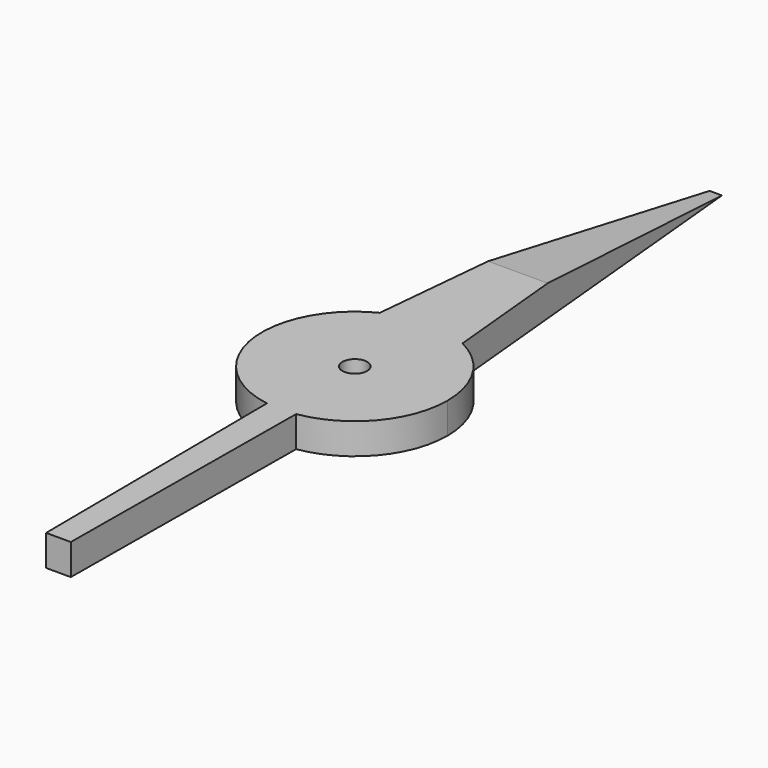
from build123d import *

# Parameters (mm, degrees)
F0_R     = 2
F1_DEPTH = 5
F2_SIZE2 = 39.99999
F2_SIZE  = 4.99999


# Not quite as in the source:
# - a fillet or chamfer is up to 0.001 mm smaller than in the source, because OpenCascade refuses the exact size


with BuildPart() as f1:
    # F0 (on Top) → F1 (new body)
    with BuildSketch(Plane.XY):
        with BuildLine():
            Line((1, 72.995454073), (0, 72.995454073))
            Line((0, 72.995454073), (-1, 72.995454073))
            Line((-1, 72.995454073), (-6.690328202, 13.4253308544))
            ThreePointArc((-6.690328202, 13.4253308544), (0, 15), (6.690328202, 13.4253308544))
            Line((6.690328202, 13.4253308544), (1, 72.995454073))
        make_face()
        with BuildLine():
            ThreePointArc((15, 0), (12.7545074979, 7.8944625204), (6.690328202, 13.4253308544))
            Line((6.690328202, 13.4253308544), (2.3585444492, -14.813415139))
            ThreePointArc((2.3585444492, -14.813415139), (11.4100430923, -9.7370897413), (15, 0))
        make_face()
        with BuildLine():
            Line((2.3585444492, -14.813415139), (6.690328202, 13.4253308544))
            ThreePointArc((6.690328202, 13.4253308544), (0, 15), (-6.690328202, 13.4253308544))
            Line((-6.690328202, 13.4253308544), (-2.3585444492, -14.813415139))
            ThreePointArc((-2.3585444492, -14.813415139), (0, -15), (2.3585444492, -14.813415139))
        make_face()
        Circle(F0_R, mode=Mode.SUBTRACT)
        with BuildLine():
            Line((-2.3585444492, -14.813415139), (-6.690328202, 13.4253308544))
            ThreePointArc((-6.690328202, 13.4253308544), (-14.8265713462, -2.2743751044), (-2.3585444492, -14.813415139))
        make_face()
        with BuildLine():
            Line((2, -59.9238947034), (2.3585444492, -14.813415139))
            ThreePointArc((2.3585444492, -14.813415139), (0, -15), (-2.3585444492, -14.813415139))
            Line((-2.3585444492, -14.813415139), (-2, -59.9238947034))
            Line((-2, -59.9238947034), (0, -59.9238947034))
            Line((0, -59.9238947034), (2, -59.9238947034))
        make_face()
    extrude(amount=F1_DEPTH)

    # F2 (size 5 and 40 in the source; OpenCascade refuses exactly that, so slightly less here)
    f2_edges = [f1.edges().sort_by_distance(p)[0] for p in [
        (0, 72.995454, 5),
    ]]
    f2_side = f1.faces().sort_by_distance((0, 72.995454, 2.5))[0]
    chamfer(f2_edges, length=F2_SIZE, length2=F2_SIZE2, reference=f2_side)


solid = f1.part
